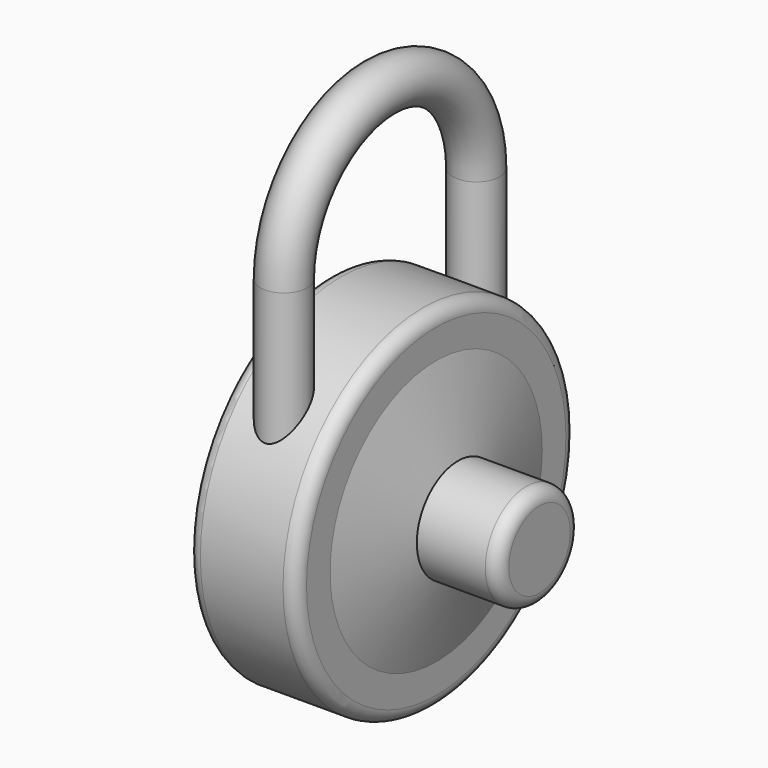
from build123d import *

# Parameters (mm, degrees)
F0_R     = 20.4558961716
F1_DEPTH = 12.7
F3_R     = 2.7480657839
F7_R     = 15.4880716028
F8_DEPTH = 2.54
F8_TAPER = 75
F9_DEPTH = 9.525
F10_R    = 1.524
F11_R    = 1.524


with BuildPart() as f1:
    # F0 (on Right) → F1 (new body)
    with BuildSketch(Plane.YZ):
        Circle(F0_R)
    extrude(amount=F1_DEPTH)

    # F6: sweep along a path in F5
    with BuildLine(Plane.YZ.offset(6.35)) as f6_path:
        Line((14.0403462574, 0), (14.0403462574, 27.4430233985))
        ThreePointArc((14.0403462574, 27.4430233985), (0, 41.4833696559), (-14.0403462574, 27.4430233985))
        Line((-14.0403462574, 27.4430233985), (-14.0403462574, 0))
    # F3 (on Top) → F6 (sweep)
    with BuildSketch(Plane.XY):
        with Locations((6.1434661038, 14.0403462574)):
            Circle(F3_R)
    sweep(path=f6_path.line)

    # F11
    f11_edges = [f1.edges().sort_by_distance(p)[0] for p in [
        (0, -20.455896, 0),
        (12.7, -20.455896, 0),
    ]]
    fillet(f11_edges, radius=F11_R)


with BuildPart() as f8:
    # F7 (on face) → F8 (new body)
    with BuildSketch(Plane.YZ.offset(12.7)):
        Circle(F7_R)
    extrude(amount=F8_DEPTH, taper=F8_TAPER)


with BuildPart() as f9:
    # F9 (new): a face of the model
    f9_faces = [f8.part.faces().sort_by_distance(p)[0] for p in [
        (15.24, 0, 0),
    ]]
    extrude(f9_faces, amount=F9_DEPTH)

    # F10
    f10_edges = [f9.edges().sort_by_distance(p)[0] for p in [
        (24.765, -6.008663, 0),
    ]]
    fillet(f10_edges, radius=F10_R)


solid = Compound([f1.part, f8.part, f9.part])
